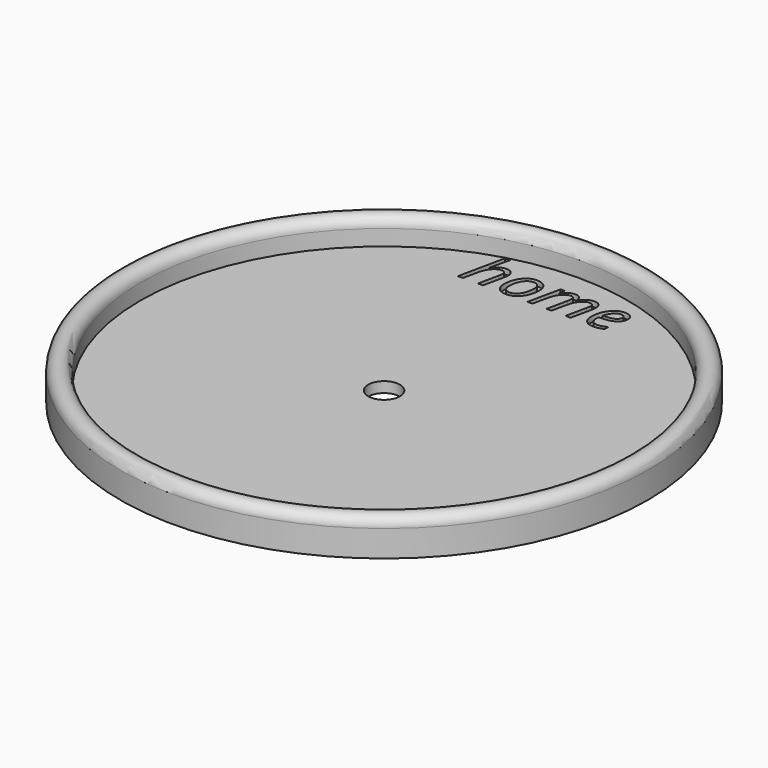
from build123d import *

# Parameters (mm, degrees)
F2_R         = 3
F3_DEPTH     = 25
F4_TEXT_SIZE = 11.5704313362
F5_DEPTH     = 1


# Not quite as in the source:
# - Text() gives the source's letters only with a copy of the font that has no kerning and outlines rounded to 1/6400 em; it was checked with that copy


with BuildPart() as f1:
    # F0 (on Front) → F1 (revolve)
    with BuildSketch(Plane.XZ):
        with BuildLine():
            Line((0, 2), (0, 0))
            Line((0, 0), (50, 0))
            Line((50, 0), (50, 5))
            ThreePointArc((50, 5), (48.0768658221, 6.9231341779), (46.1537316442, 5))
            Line((46.1537316442, 5), (46.1537316442, 2))
            Line((46.1537316442, 2), (0, 2))
        make_face()
    revolve(axis=Axis((0, 0, -0.093515031), (0, 0, -1)))

    # F2 (on face) → F3 (cut)
    with BuildSketch(Plane.XY.offset(2)):
        Circle(F2_R)
    extrude(amount=-F3_DEPTH, mode=Mode.SUBTRACT)

    # F4 (on face) → F5 (cut)
    with BuildSketch(Plane.XY.offset(2)):
        with Locations((-14.6836005176, 35.4249613048)):
            Text('home', F4_TEXT_SIZE, font='Open Sans', font_style=FontStyle.ITALIC, text_align=(TextAlign.LEFT, TextAlign.BOTTOM))
    extrude(amount=-F5_DEPTH, mode=Mode.SUBTRACT)


solid = f1.part
